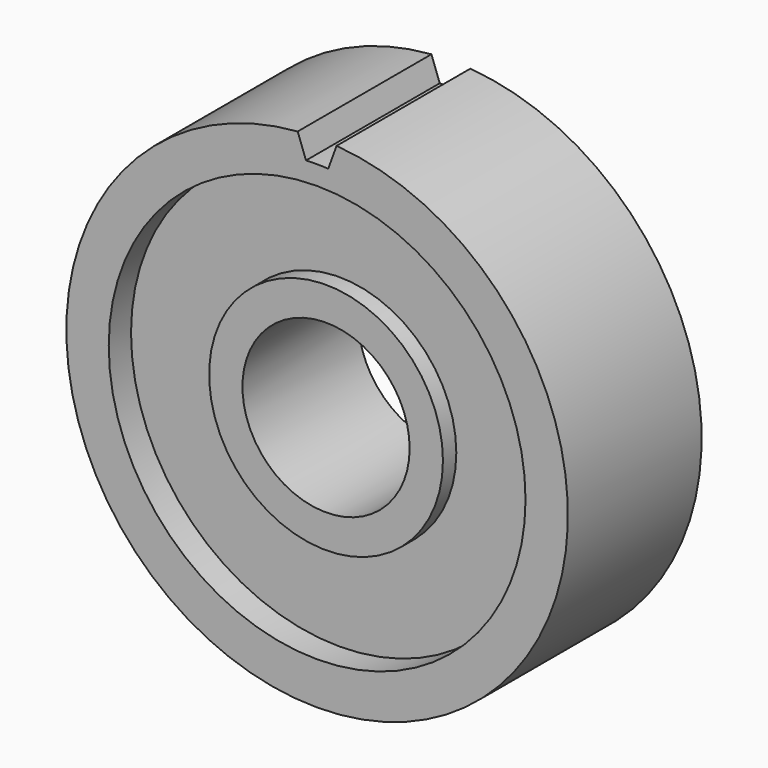
from build123d import *

# Parameters (mm, degrees)
F0_R     = 23.7453835504
F0_R_2   = 13.3203594212
F1_DEPTH = 6.35
F2_DEPTH = 9.525
F0_R_3   = 9.525
F3_DEPTH = 8.255
F4_DEPTH = 9.525
F5_DEPTH = 9.525


# Not quite as in the source:
# - a feature names something its author has since deleted; it is built from what else it names


with BuildPart() as f1:
    # F0 (on Front) → F1 (new body, symmetric)
    with BuildSketch(Plane.XZ):
        Circle(F0_R)
        Circle(F0_R_2, mode=Mode.SUBTRACT)
    extrude(amount=F1_DEPTH, both=True)

    # F0 (on Front) → F2 (join, symmetric)
    with BuildSketch(Plane.XZ):
        with BuildLine():
            ThreePointArc((25.9205484169, 0), (18.7722391675, 17.8739437974), (1.27, 25.8894173405))
            ThreePointArc((1.27, 25.8894173405), (0, 25.9205484169), (-1.27, 25.8894173405))
            ThreePointArc((-1.27, 25.8894173405), (-17.8739437974, -18.7722391675), (25.9205484169, 0))
        make_face()
        Circle(F0_R, mode=Mode.SUBTRACT)
    extrude(amount=F2_DEPTH, both=True)

    # F0 (on Front) → F3 (join, symmetric)
    with BuildSketch(Plane.XZ):
        Circle(F0_R_2)
        Circle(F0_R_3, mode=Mode.SUBTRACT)
    extrude(amount=F3_DEPTH, both=True)

    # F0 (on Front) → F4 (join, symmetric)
    with BuildSketch(Plane.XZ):
        with BuildLine():
            Line((1.27, 25.8894173405), (2.2161464291, 28.48893329))
            ThreePointArc((2.2161464291, 28.48893329), (0, 28.575), (-2.2161464291, 28.48893329))
            Line((-2.2161464291, 28.48893329), (-1.27, 25.8894173405))
            ThreePointArc((-1.27, 25.8894173405), (0, 25.9205484169), (1.27, 25.8894173405))
        make_face()
        with BuildLine():
            ThreePointArc((-2.2161464291, 28.48893329), (-19.406239213, -20.9744726896), (28.575, 0))
            ThreePointArc((28.575, 0), (20.9744726896, 19.406239213), (2.2161464291, 28.48893329))
            Line((2.2161464291, 28.48893329), (1.27, 25.8894173405))
            ThreePointArc((1.27, 25.8894173405), (18.7722391675, 17.8739437974), (25.9205484169, 0))
            ThreePointArc((25.9205484169, 0), (-17.8739437974, -18.7722391675), (-1.27, 25.8894173405))
            Line((-1.27, 25.8894173405), (-2.2161464291, 28.48893329))
        make_face()
    extrude(amount=F4_DEPTH, both=True)

    # F0 (on Front) → F5 (cut, symmetric)
    with BuildSketch(Plane.XZ):
        with BuildLine():
            Line((1.27, 25.8894173405), (2.2161464291, 28.48893329))
            ThreePointArc((2.2161464291, 28.48893329), (0, 28.575), (-2.2161464291, 28.48893329))
            Line((-2.2161464291, 28.48893329), (-1.27, 25.8894173405))
            ThreePointArc((-1.27, 25.8894173405), (0, 25.9205484169), (1.27, 25.8894173405))
        make_face()
    extrude(amount=F5_DEPTH, both=True, mode=Mode.SUBTRACT)


solid = f1.part
